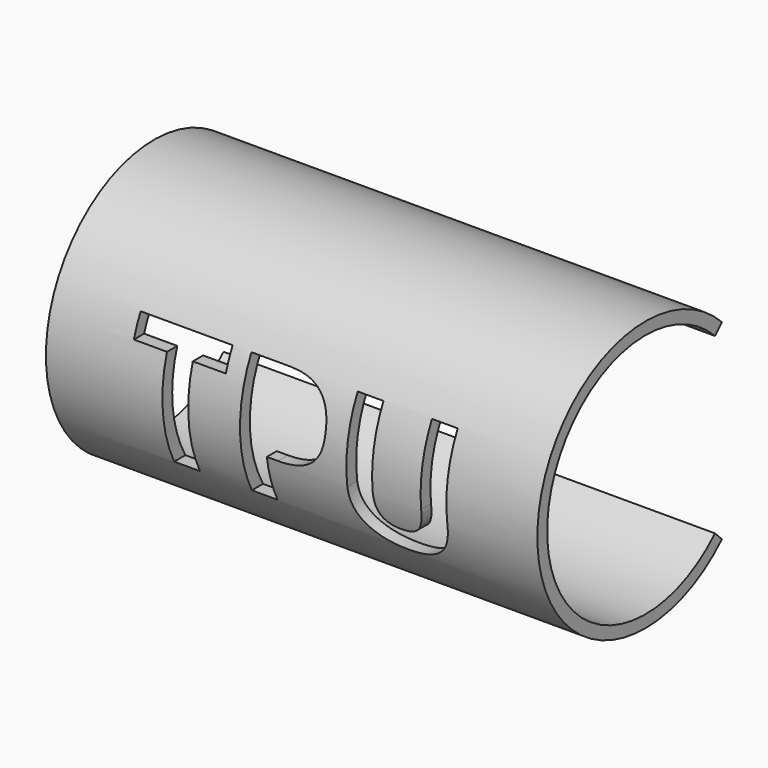
from build123d import *

# Parameters (mm, degrees)
F1_DEPTH     = 50.8
F3_TEXT_SIZE = 17.6388888889
F4_DEPTH     = 35.2792817332


# Not quite as in the source:
# - Text() gives the source's letters only with a copy of the font that has no kerning and outlines rounded to 1/6400 em; it was checked with that copy


with BuildPart() as f1:
    # F0 (on Right) → F1 (new body)
    with BuildSketch(Plane.YZ):
        with BuildLine():
            ThreePointArc((8.9802561211, -8.9802561211), (-12.7, 0), (8.9802561211, 8.9802561211))
            Line((8.9802561211, 8.9802561211), (9.8782817332, 9.8782817332))
            ThreePointArc((9.8782817332, 9.8782817332), (-13.97, 0), (9.8782817332, -9.8782817332))
            Line((9.8782817332, -9.8782817332), (8.9802561211, -8.9802561211))
        make_face()
    extrude(amount=F1_DEPTH)

    # F3 (on offset) → F4 (cut, through all)
    with BuildSketch(Plane.XZ.offset(25.4)):
        with Locations((8.2654730903, -6.35)):
            Text('TPU', F3_TEXT_SIZE, font='Open Sans', font_style=FontStyle.BOLD, text_align=(TextAlign.LEFT, TextAlign.BOTTOM))
        with BuildLine():
            Line((22.7348741319, 4.0541883681), (22.7348741319, 0.3169487847))
            Line((22.7348741319, 0.3169487847), (23.6140625, 0.3169487847))
            add(Edge.make_bspline(
                [(23.6140625, 0.3169487847), (24.8432725694, 0.3169487847), (25.4551215278, 0.8033962674)],
                knots=[0, 0, 0, 1, 1, 1], degree=2))
            add(Edge.make_bspline(
                [(25.4551215278, 0.8033962674), (26.0669704861, 1.28984375), (26.0669704861, 2.2186414931)],
                knots=[0, 0, 0, 1, 1, 1], degree=2))
            add(Edge.make_bspline(
                [(26.0669704861, 2.2186414931), (26.0669704861, 3.1584635417), (25.5543402778, 3.6063259549)],
                knots=[0, 0, 0, 1, 1, 1], degree=2))
            add(Edge.make_bspline(
                [(25.5543402778, 3.6063259549), (25.0417100694, 4.0541883681), (23.9475477431, 4.0541883681)],
                knots=[0, 0, 0, 1, 1, 1], degree=2))
            Line((23.9475477431, 4.0541883681), (22.7348741319, 4.0541883681))
        make_face()
    extrude(amount=-F4_DEPTH, mode=Mode.SUBTRACT)


solid = f1.part
